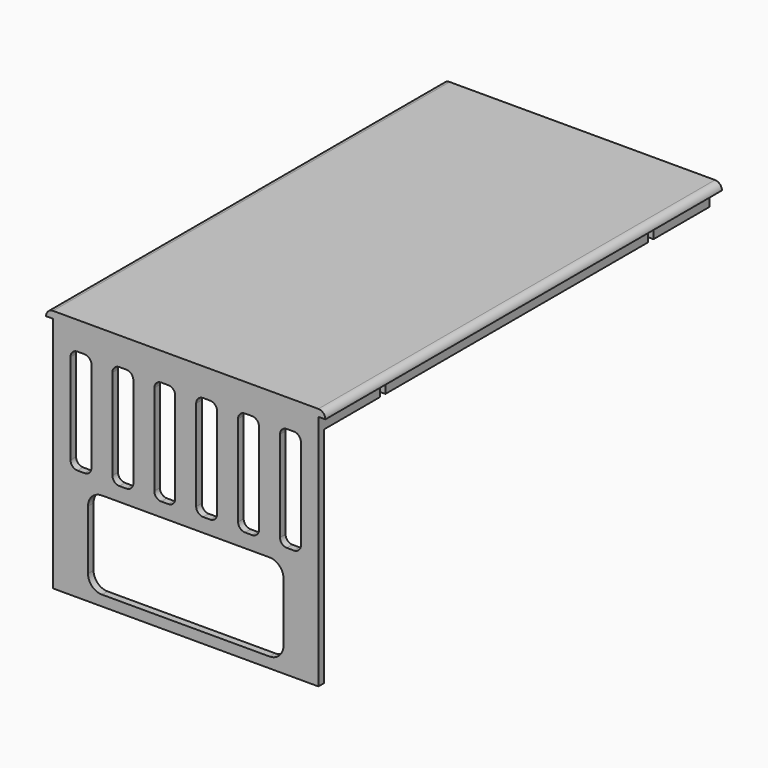
from build123d import *

# Parameters (mm, degrees)
F0_W      = 76
F0_H      = 68
F0_W_2    = 56
F0_H_2    = 25
F0_W_3    = 6
F0_H_3    = 30
F1_DEPTH  = 2
F2_W      = 80
F2_H      = 142
F3_DEPTH  = 2
F4_R      = 1.99999
F6_DEPTH  = 4
F7_R      = 4
F8_R      = 2
F9_W      = 2
F9_H      = 4
F10_DEPTH = 100


# Not quite as in the source:
# - a fillet or chamfer is up to 0.001 mm smaller than in the source, because OpenCascade refuses the exact size


with BuildPart() as f1:
    # F0 (on Front) → F1 (new body)
    with BuildSketch(Plane.XZ):
        with Locations((-2, -1)):
            Rectangle(F0_W, F0_H)
        with Locations((-2, -19.5)):
            Rectangle(F0_W_2, F0_H_2, mode=Mode.SUBTRACT)
        with Locations((-32, 12)):
            Rectangle(F0_W_3, F0_H_3, mode=Mode.SUBTRACT)
        with Locations((-20, 12)):
            Rectangle(F0_W_3, F0_H_3, mode=Mode.SUBTRACT)
        with Locations((-8, 12)):
            Rectangle(F0_W_3, F0_H_3, mode=Mode.SUBTRACT)
        with Locations((4, 12)):
            Rectangle(F0_W_3, F0_H_3, mode=Mode.SUBTRACT)
        with Locations((16, 12)):
            Rectangle(F0_W_3, F0_H_3, mode=Mode.SUBTRACT)
        with Locations((28, 12)):
            Rectangle(F0_W_3, F0_H_3, mode=Mode.SUBTRACT)
    extrude(amount=F1_DEPTH)

    # F2 (on face) → F3 (join)
    with BuildSketch(Plane.XY.offset(33)):
        with Locations((-2, 69)):
            Rectangle(F2_W, F2_H)
    extrude(amount=F3_DEPTH)

    # F4 (radius 2 in the source; OpenCascade refuses exactly that, so slightly less here)
    f4_edges = [f1.edges().sort_by_distance(p)[0] for p in [
        (38, 69, 35),
        (-42, 69, 35),
    ]]
    fillet(f4_edges, radius=F4_R)

    # F5 (on face) → F6 (join)
    with BuildSketch(Plane(origin=(0, 0, 33), x_dir=(1, 0, 0), z_dir=(0, 0, -1))):
        Polygon((-38, 0), (-40, 0), (-40, -138), (36, -138), (36, 0), (34, 0), (34, -136), (-38, -136), align=None)
    extrude(amount=F6_DEPTH)

    # F7
    f7_edges = [f1.edges().sort_by_distance(p)[0] for p in [
        (-30, -1, -7),
        (26, -1, -7),
        (-30, -1, -32),
        (26, -1, -32),
    ]]
    fillet(f7_edges, radius=F7_R)

    # F8
    f8_edges = [f1.edges().sort_by_distance(p)[0] for p in [
        (-35, -1, 27),
        (-29, -1, 27),
        (-35, -1, -3),
        (-29, -1, -3),
        (-23, -1, 27),
        (-17, -1, 27),
        (-23, -1, -3),
        (-17, -1, -3),
        (-11, -1, -3),
        (-11, -1, 27),
        (-5, -1, 27),
        (-5, -1, -3),
        (1, -1, -3),
        (7, -1, -3),
        (7, -1, 27),
        (1, -1, 27),
        (13, -1, 27),
        (19, -1, 27),
        (19, -1, -3),
        (13, -1, -3),
        (25, -1, -3),
        (31, -1, -3),
        (25, -1, 27),
        (31, -1, 27),
    ]]
    fillet(f8_edges, radius=F8_R)

    # F9 (on face) → F10 (cut, symmetric)
    with BuildSketch(Plane(origin=(-40, 0, 0), x_dir=(0, -1, 0), z_dir=(-1, 0, 0))):
        with Locations((-117, 31)):
            Rectangle(F9_W, F9_H)
        with Locations((-21, 31)):
            Rectangle(F9_W, F9_H)
    extrude(amount=F10_DEPTH, both=True, mode=Mode.SUBTRACT)


solid = f1.part
